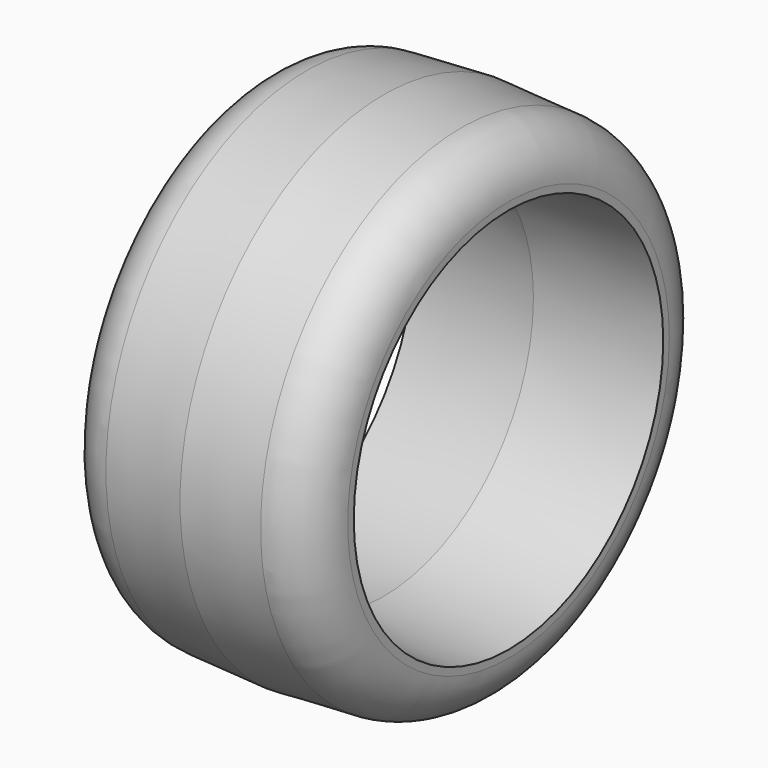
from build123d import *

# Parameters (mm, degrees)
F2_R     = 25.9753807736
F2_R_2   = 19.05
F3_DEPTH = 12.7
F3_TAPER = 3
F4_R     = 5.08


# Not quite as in the source:
# - two fillets or chamfers of one size are made in one step


with BuildPart() as f3:
    # F2 (on offset) → F3 (new body, symmetric)
    with BuildSketch(Plane.YZ.offset(50.8)):
        Circle(F2_R)
        Circle(F2_R_2, mode=Mode.SUBTRACT)
    extrude(amount=F3_DEPTH, both=True, taper=F3_TAPER)

    # F4
    f4_edges = [f3.edges().sort_by_distance(p)[0] for p in [
        (63.5, -25.309802, 0),
        (38.1, -25.309802, 0),
    ]]
    fillet(f4_edges, radius=F4_R)


solid = f3.part
